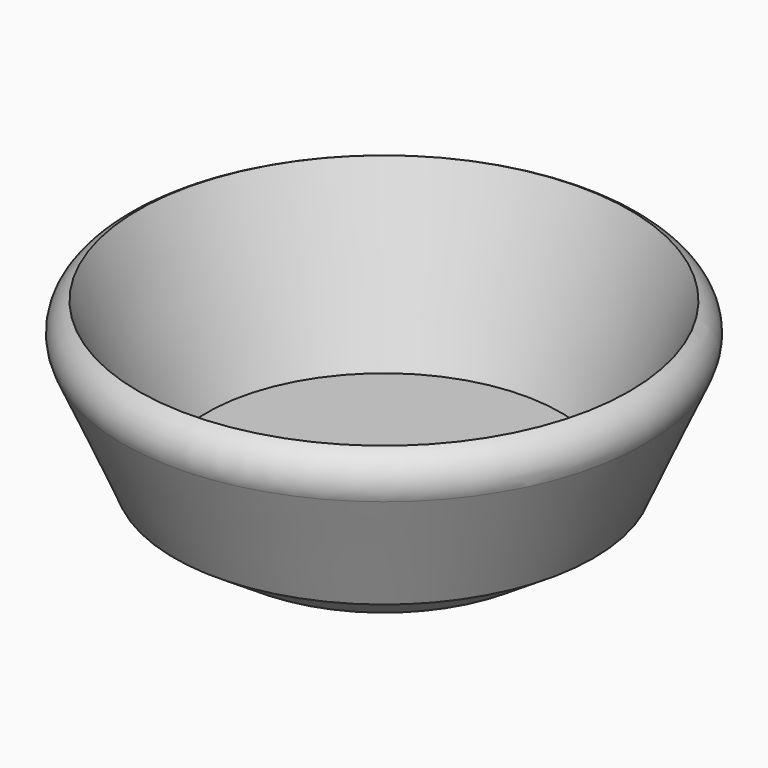
from build123d import *

# Parameters (mm, degrees)
F3_SIZE = 2.54


# Not quite as in the source:
# - a fillet or chamfer that OpenCascade refuses, or shapes differently, is made with other operations: its cross-section is extruded or revolved along the edge and cut away or added


with BuildPart() as f1:
    # F0 (on Front) → F1 (revolve)
    with BuildSketch(Plane.XZ):
        Polygon((0, 2.484759083), (0, 0), (12.7, 0), (18.2904321501, 12.7), (16.0741669896, 12.7), (11.577504687, 2.484759083), align=None)
    revolve(axis=Axis((0, 0, 10.5566112325), (0, 0, 1)))

    # F2: fillet of radius 2.0499963011 on 1 edges, made by hand

    # F2_s1 → F2_t2 (revolve, cut)
    with BuildSketch(Plane.XZ):
        with BuildLine():
            ThreePointArc((17.1048272979, 10.0066158002), (17.1431716206, 11.5651790127), (16.0741669896, 12.7))
            Line((16.0741669896, 12.7), (18.2904321501, 12.7))
            Line((18.2904321501, 12.7), (17.1048272979, 10.0066158002))
        make_face()
    revolve(axis=Axis((0, 0, 12.7), (0, 0, 1)), mode=Mode.SUBTRACT)

    # F3
    f3_edges = [f1.edges().sort_by_distance(p)[0] for p in [
        (-12.7, 0, 0),
    ]]
    chamfer(f3_edges, length=F3_SIZE)


solid = f1.part
